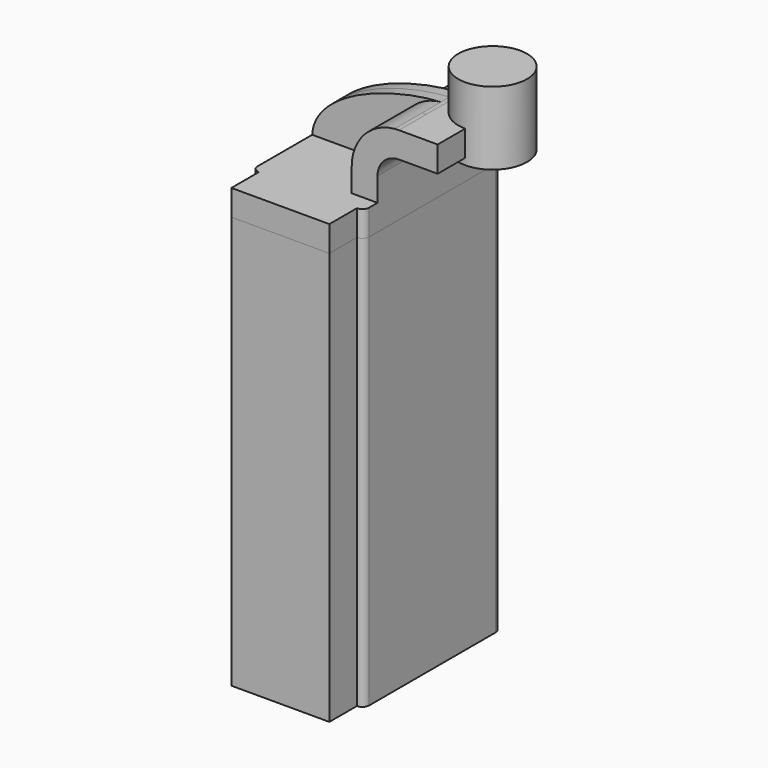
from build123d import *

# Parameters (mm, degrees)
F1_DEPTH = 63.5
F0_W     = 25.4
F0_H     = 19.05
F2_DEPTH = 25.4
F3_DEPTH = 7.9375
F5_R     = 5.08
F6_DEPTH = 25.4
F7_DEPTH = 25.4
F8_DEPTH = 304.8


with BuildPart() as f1:
    # F0 (on Front) → F1 (new body, symmetric)
    with BuildSketch(Plane.XZ):
        Polygon((22.225, 9.525), (-41.275, 9.525), (-41.275, -9.525), (41.275, -9.525), (41.275, 9.525), align=None)
    extrude(amount=F1_DEPTH, both=True)

    # F0 (on Front) → F2 (join, symmetric)
    with BuildSketch(Plane.XZ):
        with BuildLine():
            Line((22.225, 27.0002), (22.225, 9.525))
            Line((22.225, 9.525), (41.275, 9.525))
            Line((41.275, 9.525), (41.275, 27.0002))
            ThreePointArc((41.275, 27.0002), (45.9246798487, 38.2255201513), (57.15, 42.8752))
            Line((57.15, 42.8752), (60.325, 42.8752))
            Line((60.325, 42.8752), (60.325, 61.9252))
            Line((60.325, 61.9252), (57.15, 61.9252))
            add(Edge.make_bspline(
                [(53.8854342407, 61.7722898912), (54.9842067368, 61.8365871986), (56.0728453275, 61.8876096574), (57.15, 61.9252)],
                knots=[108.5245810491, 108.5245810491, 108.5245810491, 108.5245810491, 111.5045361635, 111.5045361635, 111.5045361635, 111.5045361635], degree=3))
            ThreePointArc((53.8854342407, 61.7722898912), (31.3258777096, 50.5133948686), (22.225, 27.0002))
        make_face()
        with Locations((73.025, 52.4002)):
            Rectangle(F0_W, F0_H)
    extrude(amount=F2_DEPTH, both=True)

    # F0 (on Front) → F3 (join, symmetric)
    with BuildSketch(Plane.XZ):
        with BuildLine():
            add(Edge.make_bspline(
                [(-41.275, 9.525), (-39.5856284224, 39.4828766469), (13.870125209, 59.4306981306), (53.8854342407, 61.7722898912)],
                knots=[0, 0, 0, 0, 108.5245810491, 108.5245810491, 108.5245810491, 108.5245810491], degree=3))
            Line((-41.275, 9.525), (22.225, 9.525))
            Line((22.225, 9.525), (22.225, 27.0002))
            ThreePointArc((22.225, 27.0002), (31.3258777096, 50.5133948686), (53.8854342407, 61.7722898912))
        make_face()
    extrude(amount=F3_DEPTH, both=True)

    # F0 (on Front) → F4 (revolve)
    with BuildSketch(Plane.XZ):
        Polygon((85.725, 66.675), (85.725, 61.9252), (85.725, 42.8752), (85.725, 38.1), (111.125, 38.1), (111.125, 66.675), align=None)
    revolve(axis=Axis((85.725, 0, 52.3875), (0, 0, 1)))

    # F5
    f5_edges = [f1.edges().sort_by_distance(p)[0] for p in [
        (41.275, -63.5, 0),
        (-41.275, -63.5, 0),
        (41.275, 63.5, 0),
        (-41.275, 63.5, 0),
    ]]
    fillet(f5_edges, radius=F5_R)

    # F6 (add): a face of the model
    f6_faces = [f1.faces().sort_by_distance(p)[0] for p in [
        (85.725, 0, 66.675),
    ]]
    extrude(f6_faces, amount=F6_DEPTH)

    # F7 (add): faces of the model
    f7_faces = [f1.faces().sort_by_distance(p)[0] for p in [
        (48.8772671015, -25.4, 41.5257592525),
        (0, -63.5, 0),
    ]]
    extrude(f7_faces, amount=F7_DEPTH)

    # F8 (add): a face of the model
    f8_faces = [f1.faces().sort_by_distance(p)[0] for p in [
        (0, -11.3906341446, -9.525),
    ]]
    extrude(f8_faces, amount=F8_DEPTH)


solid = f1.part
